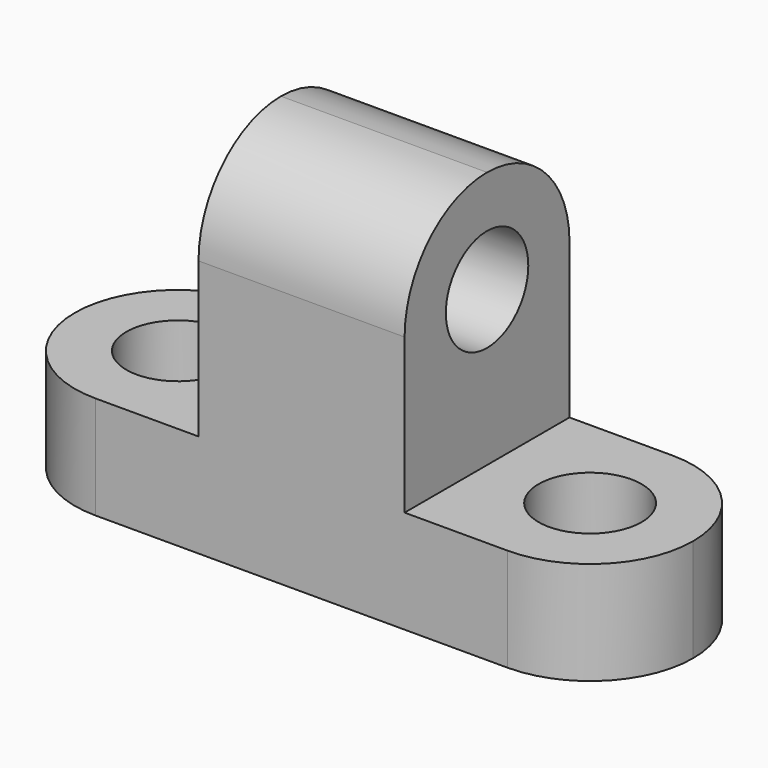
from build123d import *

# Parameters (mm, degrees)
F0_W      = 25.4
F0_H      = 44.45
F1_DEPTH  = 25.4
F2_R      = 12.69999
F4_R      = 6.35
F5_DEPTH  = 25.4
F6_W      = 25.4
F6_H      = 25.4
F7_DEPTH  = 12.7
F8_R      = 12.69999
F9_R      = 12.69999
F10_R     = 6.35
F11_DEPTH = 12.7
F12_R     = 6.35
F13_DEPTH = 12.7


# Not quite as in the source:
# - a fillet or chamfer is up to 0.001 mm smaller than in the source, because OpenCascade refuses the exact size


with BuildPart() as f1:
    # F0 (on Front) → F1 (new body)
    with BuildSketch(Plane.XZ):
        with Locations((12.7, 22.225)):
            Rectangle(F0_W, F0_H)
    extrude(amount=-F1_DEPTH)

    # F2 (radius 12.7 in the source; OpenCascade refuses exactly that, so slightly less here)
    f2_edges = [f1.edges().sort_by_distance(p)[0] for p in [
        (12.7, 0, 44.45),
        (12.7, 25.4, 44.45),
    ]]
    fillet(f2_edges, radius=F2_R)

    # F4 (on Right) → F5 (cut)
    with BuildSketch(Plane.YZ):
        with Locations((12.7, 31.75)):
            Circle(F4_R)
    extrude(amount=F5_DEPTH, mode=Mode.SUBTRACT)

    # F6 (on Top) → F7 (join)
    with BuildSketch(Plane.XY):
        with Locations((-12.7, 12.7)):
            Rectangle(F6_W, F6_H)
        with Locations((38.1, 12.7)):
            Rectangle(F6_W, F6_H)
    extrude(amount=F7_DEPTH)

    # F8 (radius 12.7 in the source; OpenCascade refuses exactly that, so slightly less here)
    f8_edges = [f1.edges().sort_by_distance(p)[0] for p in [
        (-25.4, 25.4, 6.35),
        (-25.4, 0, 6.35),
    ]]
    fillet(f8_edges, radius=F8_R)

    # F9 (radius 12.7 in the source; OpenCascade refuses exactly that, so slightly less here)
    f9_edges = [f1.edges().sort_by_distance(p)[0] for p in [
        (50.8, 0, 6.35),
        (50.8, 25.4, 6.35),
    ]]
    fillet(f9_edges, radius=F9_R)

    # F10 (on Top) → F11 (cut)
    with BuildSketch(Plane.XY):
        with Locations((-12.7, 12.7)):
            Circle(F10_R)
    extrude(amount=F11_DEPTH, mode=Mode.SUBTRACT)

    # F12 (on Top) → F13 (cut)
    with BuildSketch(Plane.XY):
        with Locations((38.1, 12.7)):
            Circle(F12_R)
    extrude(amount=F13_DEPTH, mode=Mode.SUBTRACT)


solid = f1.part
